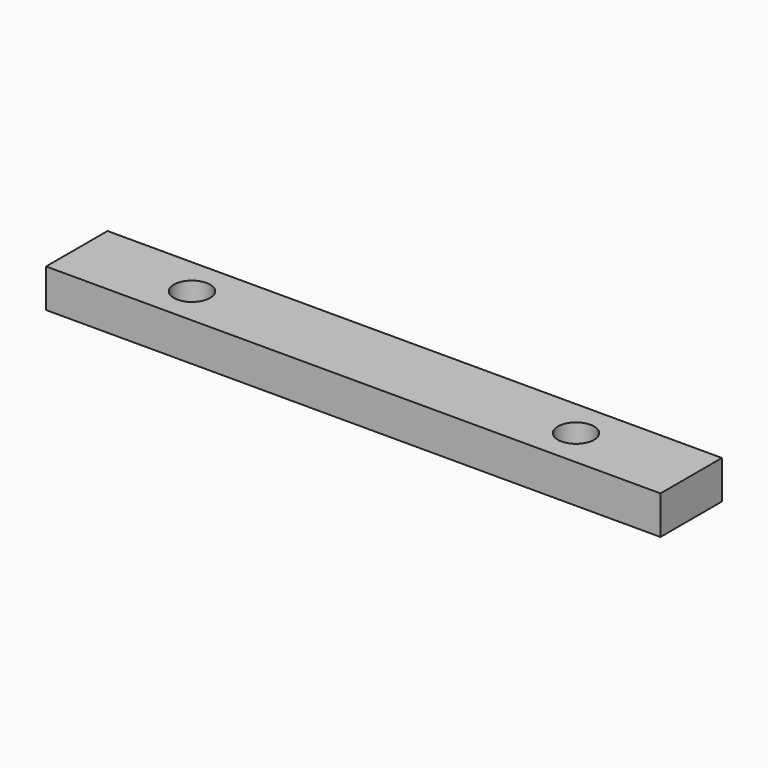
from build123d import *

# Parameters (mm, degrees)
F0_W     = 101.6
F0_H     = 12.7
F0_R     = 3.0003539725
F1_DEPTH = 6.35


# Not quite as in the source:
# - a length typed as a fraction of an inch, garbled in the dataset ("3 / 203.2 mm" for 3/8 in), is restored


with BuildPart() as f1:
    # F0 (on Top) → F1 (new body)
    with BuildSketch(Plane.XY):
        with Locations((50.8, 6.35)):
            Rectangle(F0_W, F0_H)
        with Locations((19.05, 6.35)):
            Circle(F0_R, mode=Mode.SUBTRACT)
        with Locations((82.55, 6.35)):
            Circle(F0_R, mode=Mode.SUBTRACT)
    extrude(amount=F1_DEPTH)


solid = f1.part
